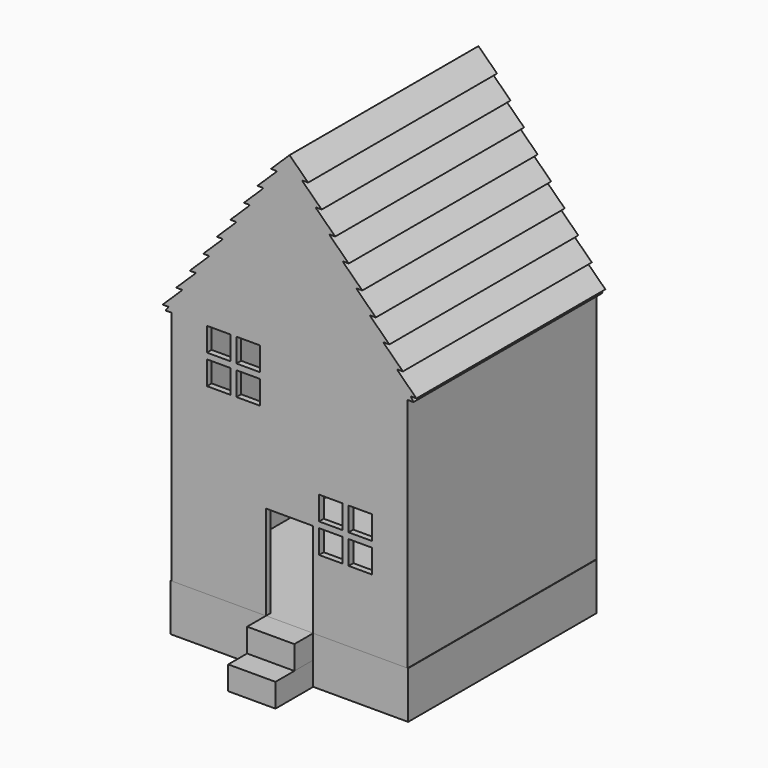
from build123d import *

# Parameters (mm, degrees)
F0_W      = 508
F0_H      = 508
F0_W_2    = 482.6000034809
F0_H_2    = 482.6000034809
F1_DEPTH  = 508
F3_DEPTH  = 508
F4_W      = 50.8
F4_H      = 50.8
F5_DEPTH  = 734.06
F6_W      = 101.6
F6_H      = 203.2
F7_DEPTH  = 25.4
F10_W     = 511.2411379814
F10_H     = 506.5713822842
F11_DEPTH = 101.6
F12_W     = 101.6
F12_H     = 50.8
F13_DEPTH = 101.6
F14_W     = 101.6
F14_H     = 50.8
F15_DEPTH = 50.8


# Not quite as in the source:
# - the program builds the solid bodies; features that only make, move or delete a surface that nothing else refers to are left out


with BuildPart() as f1:
    # F0 (on Top) → F1 (new body)
    with BuildSketch(Plane.XY):
        Rectangle(F0_W, F0_H)
        Rectangle(F0_W_2, F0_H_2, mode=Mode.SUBTRACT)
    extrude(amount=F1_DEPTH)

    # F2 (on face) → F3 (join)
    with BuildSketch(Plane.XZ.offset(254)):
        Polygon((-260.3633201527, 517.0523997819), (-266.7, 508), (266.7, 508), (260.3633201527, 517.0523997819), (273.0633201527, 517.0523997819), (233.0550967493, 556.0641475011), (231.231433059, 558.6693813443), (243.931433059, 558.6693813443), (203.9232096556, 597.6811290634), (202.0995459654, 600.2863629066), (214.7995459654, 600.2863629066), (174.7913225619, 639.2981106258), (172.9676588717, 641.903344469), (185.6676588717, 641.903344469), (145.6594354683, 680.9150921882), (143.835771778, 683.5203260314), (156.535771778, 683.5203260314), (116.5275483746, 722.5320737505), (114.7038846844, 725.1373075937), (127.4038846844, 725.1373075937), (87.395661281, 764.1490553129), (85.5719975907, 766.7542891561), (98.2719975907, 766.7542891561), (58.2637741873, 805.7660368753), (56.4401104971, 808.3712707185), (69.1401104971, 808.3712707185), (29.1318870937, 847.3830184376), (27.3082234034, 849.9882522808), (40.0082234034, 849.9882522808), (0, 889), (-40.0082234034, 849.9882522808), (-27.3082234034, 849.9882522808), (-29.1318870937, 847.3830184376), (-69.1401104971, 808.3712707185), (-56.4401104971, 808.3712707185), (-58.2637741873, 805.7660368753), (-98.2719975907, 766.7542891561), (-85.5719975907, 766.7542891561), (-87.395661281, 764.1490553129), (-127.4038846844, 725.1373075937), (-114.7038846844, 725.1373075937), (-116.5275483746, 722.5320737505), (-156.535771778, 683.5203260314), (-143.835771778, 683.5203260314), (-145.6594354683, 680.9150921882), (-185.6676588717, 641.903344469), (-172.9676588717, 641.903344469), (-174.7913225619, 639.2981106258), (-214.7995459654, 600.2863629066), (-202.0995459654, 600.2863629066), (-203.9232096556, 597.6811290634), (-243.931433059, 558.6693813443), (-231.231433059, 558.6693813443), (-233.0550967493, 556.0641475011), (-273.0633201527, 517.0523997819), align=None)
    extrude(amount=-F3_DEPTH)

    # F4 (on face) → F5 (cut)
    with BuildSketch(Plane.XZ.offset(254)):
        with Locations((-88.9, 482.6)):
            Rectangle(F4_W, F4_H)
        with Locations((-152.4, 419.1)):
            Rectangle(F4_W, F4_H)
        with Locations((-88.9, 419.1)):
            Rectangle(F4_W, F4_H)
        with Locations((-152.4, 482.6)):
            Rectangle(F4_W, F4_H)
        with Locations((152.4, 241.3)):
            Rectangle(F4_W, F4_H)
        with Locations((88.9, 177.8)):
            Rectangle(F4_W, F4_H)
        with Locations((152.4, 177.8)):
            Rectangle(F4_W, F4_H)
        with Locations((88.9, 241.3)):
            Rectangle(F4_W, F4_H)
    extrude(amount=-F5_DEPTH, mode=Mode.SUBTRACT)

    # F6 (on face) → F7 (cut)
    with BuildSketch(Plane.XZ.offset(254)):
        with Locations((0, 101.6)):
            Rectangle(F6_W, F6_H)
    extrude(amount=-F7_DEPTH, mode=Mode.SUBTRACT)

    # F10 (on Top) → F11 (join)
    with BuildSketch(Plane.XY):
        with Locations((-0.6510317326, -0.4706829786)):
            Rectangle(F10_W, F10_H)
    extrude(amount=-F11_DEPTH)

    # F12 (on face) → F13 (join)
    with BuildSketch(Plane.XZ.offset(253.7563741207)):
        with Locations((0, -76.2)):
            Rectangle(F12_W, F12_H)
    extrude(amount=F13_DEPTH)


with BuildPart() as f15:
    # F14 (on face) → F15 (new body)
    with BuildSketch(Plane.XZ.offset(253.7563741207)):
        with Locations((0, -25.4)):
            Rectangle(F14_W, F14_H)
    extrude(amount=F15_DEPTH)


solid = Compound([f1.part, f15.part])
